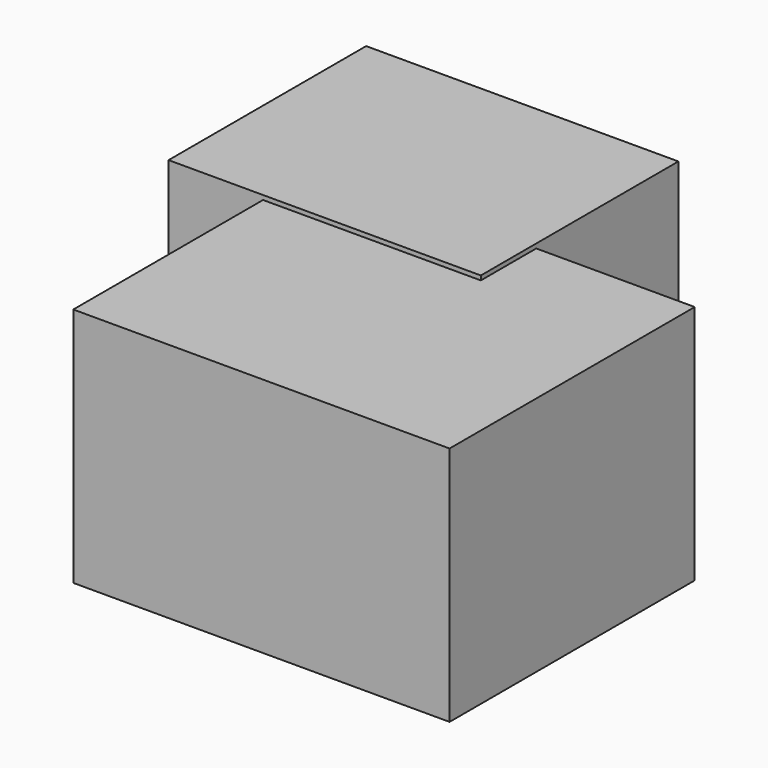
from build123d import *

# Parameters (mm, degrees)
F0_W     = 72.66
F0_H     = 57.46
F1_DEPTH = 57.03
F2_W     = 87.56
F2_H     = 71.3
F3_DEPTH = 56.01


# Not quite as in the source:
# - a feature names something its author has since deleted; it is built from what else it names


with BuildPart() as f1:
    # F0 (on Top) → F1 (new body)
    with BuildSketch(Plane.XY):
        with Locations((-52.8233502674, 43.0624267119)):
            Rectangle(F0_W, F0_H)
    extrude(amount=F1_DEPTH)

    # F2 (on Top) → F3 (join)
    with BuildSketch(Plane.XY):
        with Locations((-23.3953585339, -5.2052624285)):
            Rectangle(F2_W, F2_H)
    extrude(amount=F3_DEPTH)


solid = f1.part
